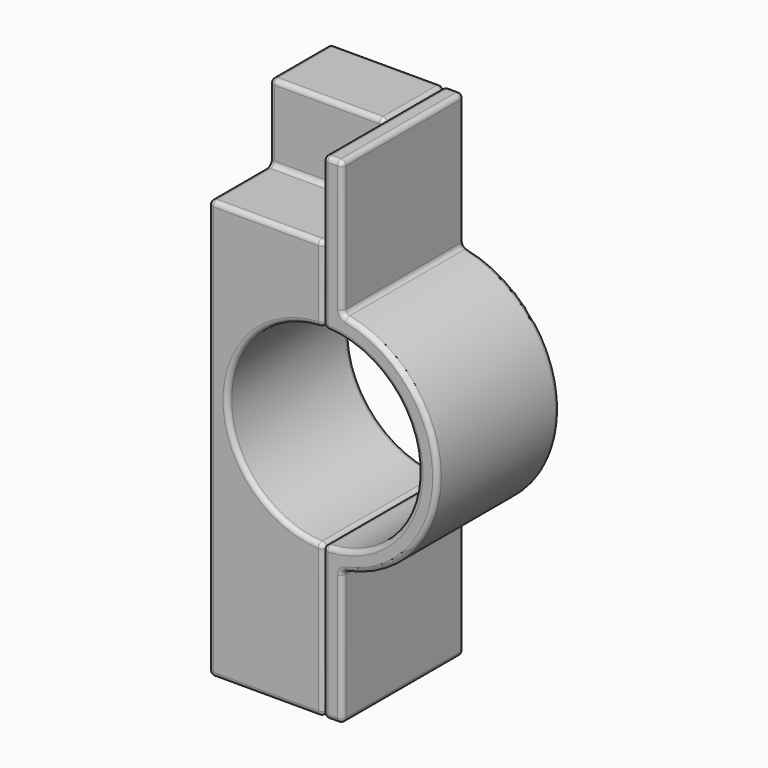
from build123d import *

# Parameters (mm, degrees)
F1_DEPTH = 12.7
F2_R     = 0.396875
F3_DEPTH = 12.7
F4_W     = 6.35
F4_H     = 6.35
F5_DEPTH = 25.4
F6_R     = 0.396875


with BuildPart() as f1:
    # F0 (on Front) → F1 (new body)
    with BuildSketch(Plane.XZ):
        with BuildLine():
            ThreePointArc((0, 7.9375), (7.9375, 0), (0, -7.9375))
            Line((0, -7.9375), (0, -20.6375))
            Line((0, -20.6375), (1.6002, -20.6375))
            Line((1.6002, -20.6375), (1.6002, -9.4025039883))
            ThreePointArc((1.6002, -9.4025039883), (9.5377, 0), (1.6002, 9.4025039883))
            Line((1.6002, 9.4025039883), (1.6002, 20.6375))
            Line((1.6002, 20.6375), (0, 20.6375))
            Line((0, 20.6375), (0, 7.9375))
        make_face()
    extrude(amount=F1_DEPTH)

    # F2
    f2_edges = [f1.edges().sort_by_distance(p)[0] for p in [
        (1.6002, -6.35, 9.402504),
        (1.6002, -6.35, -9.402504),
        (0, -6.35, 7.9375),
        (0, -6.35, -7.9375),
        (7.9375, 0, 0),
        (0, 0, -14.2875),
        (0.8001, 0, -20.6375),
        (1.6002, 0, -15.020002),
        (9.5377, 0, 0),
        (1.6002, 0, 15.020002),
        (0.8001, 0, 20.6375),
        (0, 0, 14.2875),
        (7.9375, -12.7, 0),
        (0, -12.7, -14.2875),
        (0.8001, -12.7, -20.6375),
        (1.6002, -12.7, -15.020002),
        (9.5377, -12.7, 0),
        (1.6002, -12.7, 15.020002),
        (0.8001, -12.7, 20.6375),
        (0, -12.7, 14.2875),
        (0, -6.35, -20.6375),
        (1.6002, -6.35, -20.6375),
        (1.6002, -6.35, 20.6375),
        (0, -6.35, 20.6375),
    ]]
    fillet(f2_edges, radius=F2_R)


with BuildPart() as f3:
    # F0 (on Front) → F3 (new body)
    with BuildSketch(Plane.XZ):
        with BuildLine():
            Line((0, -20.6375), (0, -7.9375))
            ThreePointArc((0, -7.9375), (-7.9375, 0), (0, 7.9375))
            Line((0, 7.9375), (0, 20.6375))
            Line((0, 20.6375), (-1.6002, 20.6375))
            Line((-1.6002, 20.6375), (-9.5377, 20.6375))
            Line((-9.5377, 20.6375), (-9.5377, 0))
            Line((-9.5377, 0), (-9.5377, -20.6375))
            Line((-9.5377, -20.6375), (-1.6002, -20.6375))
            Line((-1.6002, -20.6375), (0, -20.6375))
        make_face()
    extrude(amount=F3_DEPTH)

    # F4 (on face) → F5 (cut)
    with BuildSketch(Plane(origin=(-9.5377, 0, 0), x_dir=(0, -1, 0), z_dir=(-1, 0, 0))):
        with Locations((9.525, 17.4625)):
            Rectangle(F4_W, F4_H)
    extrude(amount=-F5_DEPTH, mode=Mode.SUBTRACT)

    # F6
    f6_edges = [f3.edges().sort_by_distance(p)[0] for p in [
        (0, -6.35, -7.9375),
        (0, -6.35, 7.9375),
        (-7.9375, 0, 0),
        (-7.9375, -12.7, 0),
        (0, 0, -14.2875),
        (0, 0, 14.2875),
        (-4.76885, 0, 20.6375),
        (-9.5377, 0, 0),
        (-4.76885, 0, -20.6375),
        (-4.76885, -12.7, -20.6375),
        (-9.5377, -12.7, -3.175),
        (-4.76885, -12.7, 14.2875),
        (0, -12.7, 11.1125),
        (0, -12.7, -14.2875),
        (-9.5377, -3.175, 20.6375),
        (-4.76885, -6.35, 20.6375),
        (0, -3.175, 20.6375),
        (-9.5377, -6.35, -20.6375),
        (0, -6.35, -20.6375),
        (-9.5377, -6.35, 17.4625),
        (-4.76885, -6.35, 14.2875),
        (0, -6.35, 17.4625),
        (-9.5377, -9.525, 14.2875),
        (0, -9.525, 14.2875),
    ]]
    fillet(f6_edges, radius=F6_R)


solid = Compound([f1.part, f3.part])
